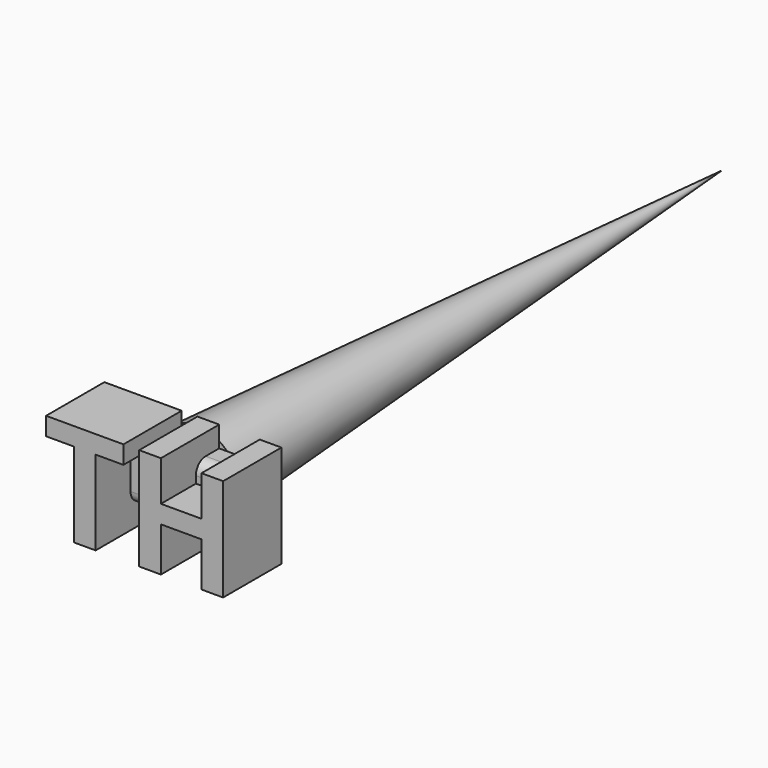
from build123d import *

# Parameters (mm, degrees)
F0_TEXT_SIZE = 15.0110810145
F1_DEPTH     = 7.62
F2_W         = 14.6301139692
F2_H         = 6.2248213084
F3_DEPTH     = 3.048
F6_R         = 1.27


# Not quite as in the source:
# - Text() gives the source's letters only with a copy of the font that has no kerning and outlines rounded to 1/6400 em; it was checked with that copy


with BuildPart() as f1:
    # F0 (on Front) → F1 (new body)
    with BuildSketch(Plane.XZ):
        with Locations((-9.9635396592, -5.434663609)):
            Text('TH', F0_TEXT_SIZE, font='Open Sans', font_style=FontStyle.BOLD, text_align=(TextAlign.LEFT, TextAlign.BOTTOM))
    extrude(amount=F1_DEPTH)

    # F2 (on Front) → F3 (join)
    with BuildSketch(Plane.XZ):
        with Locations((0.8221958692, -0.0243051195)):
            Rectangle(F2_W, F2_H)
    extrude(amount=F3_DEPTH)

    # F6
    f6_edges = [f1.edges().sort_by_distance(p)[0] for p in [
        (-2.201169, -3.048, 3.088106),
        (4.471726, -3.048, 3.088106),
        (-2.201169, -3.048, -3.136716),
        (4.471726, -3.048, -3.136716),
    ]]
    fillet(f6_edges, radius=F6_R)


with BuildPart() as f5:
    # F4 (on Top) → F5 (revolve)
    with BuildSketch(Plane.XY):
        Polygon((-4.4356729389, 0), (0, 0), (0, 68.681396544), align=None)
    revolve(axis=Axis((0, 34.340698272, 0), (0, 1, 0)))


solid = Compound([f1.part, f5.part])
